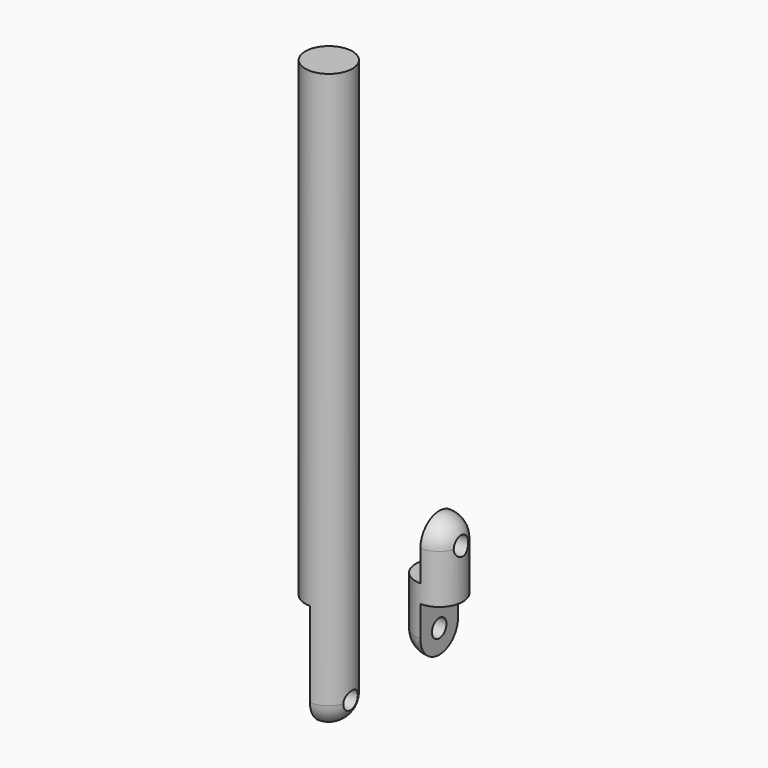
from build123d import *

# Parameters (mm, degrees)
F0_R      = 8.255
F1_DEPTH  = 203.2
F2_R      = 8.255
F3_W      = 65.5652643557
F3_H      = 67.8089395726
F4_DEPTH  = 25.4
F5_R      = 3.175
F6_DEPTH  = 25.4
F7_R      = 8.255
F8_DEPTH  = 44.45
F9_W      = 28.5546391179
F9_H      = 24.6901003341
F10_DEPTH = 25.4
F11_R     = 8.25499
F12_R     = 3.175
F13_DEPTH = 25.4
F14_W     = 34.453469107
F14_H     = 29.3156715315
F15_DEPTH = 25.4
F16_R     = 8.25499
F17_R     = 3.175
F18_DEPTH = 25.4


# Not quite as in the source:
# - a fillet or chamfer is up to 0.001 mm smaller than in the source, because OpenCascade refuses the exact size


with BuildPart() as f1:
    # F0 (on Top) → F1 (new body)
    with BuildSketch(Plane.XY):
        Circle(F0_R)
    extrude(amount=F1_DEPTH)

    # F2
    f2_edges = [f1.edges().sort_by_distance(p)[0] for p in [
        (-8.255, 0, 0),
    ]]
    fillet(f2_edges, radius=F2_R)

    # F3 (on Right) → F4 (cut)
    with BuildSketch(Plane.YZ):
        with Locations((-3.3156136051, 4.1955302137)):
            Rectangle(F3_W, F3_H)
    extrude(amount=-F4_DEPTH, mode=Mode.SUBTRACT)

    # F5 (on face) → F6 (cut)
    with BuildSketch(Plane(origin=(0, 0, 0), x_dir=(0, -1, 0), z_dir=(-1, 0, 0))):
        with Locations((0, 8.255)):
            Circle(F5_R)
    extrude(amount=-F6_DEPTH, mode=Mode.SUBTRACT)


with BuildPart() as f8:
    # F7 (on Top) → F8 (new body)
    with BuildSketch(Plane.XY):
        with Locations((0, 48.3787283301)):
            Circle(F7_R)
    extrude(amount=F8_DEPTH)

    # F9 (on Right) → F10 (cut)
    with BuildSketch(Plane.YZ):
        with Locations((48.8578211516, 37.745050167)):
            Rectangle(F9_W, F9_H)
    extrude(amount=-F10_DEPTH, mode=Mode.SUBTRACT)

    # F11 (radius 8.255 in the source; OpenCascade refuses exactly that, so slightly less here)
    f11_edges = [f8.edges().sort_by_distance(p)[0] for p in [
        (5.837166, 42.541562, 44.45),
        (5.837166, 54.215895, 44.45),
    ]]
    fillet(f11_edges, radius=F11_R)

    # F12 (on face) → F13 (cut)
    with BuildSketch(Plane(origin=(0, 0, 0), x_dir=(0, -1, 0), z_dir=(-1, 0, 0))):
        with Locations((-48.3787283301, 36.195)):
            Circle(F12_R)
    extrude(amount=-F13_DEPTH, mode=Mode.SUBTRACT)

    # F14 (on Right) → F15 (cut)
    with BuildSketch(Plane.YZ):
        with Locations((49.3318922818, 4.3921642342)):
            Rectangle(F14_W, F14_H)
    extrude(amount=F15_DEPTH, mode=Mode.SUBTRACT)

    # F16 (radius 8.255 in the source; OpenCascade refuses exactly that, so slightly less here)
    f16_edges = [f8.edges().sort_by_distance(p)[0] for p in [
        (-8.255, 48.378728, 0),
    ]]
    fillet(f16_edges, radius=F16_R)

    # F17 (on face) → F18 (cut)
    with BuildSketch(Plane.YZ):
        with Locations((48.3787283301, 8.255)):
            Circle(F17_R)
    extrude(amount=-F18_DEPTH, mode=Mode.SUBTRACT)


solid = Compound([f1.part, f8.part])
